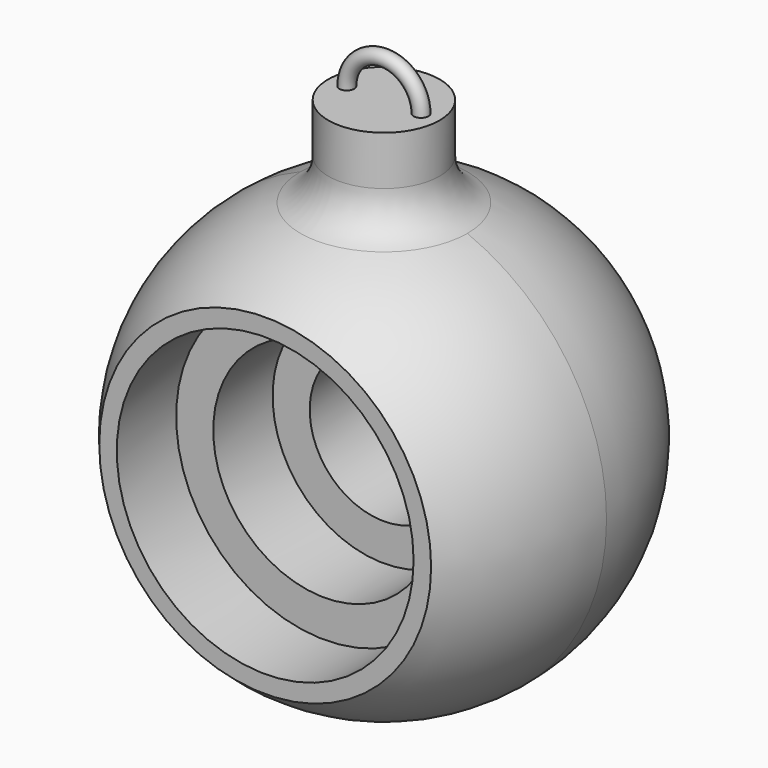
from build123d import *

# Parameters (mm, degrees)
F3_R      = 6.35
F4_DEPTH  = 63.5
F3_R_2    = 12.7
F5_DEPTH  = 50.8
F3_R_3    = 19.05
F6_DEPTH  = 38.1
F3_R_4    = 25.4
F7_DEPTH  = 25.4
F3_R_5    = 31.75
F8_DEPTH  = 12.7
F10_R     = 9.525
F11_DEPTH = 12.7
F14_R     = 1.27


# Not quite as in the source:
# - a fillet or chamfer that OpenCascade refuses, or shapes differently, is made with other operations: its cross-section is extruded or revolved along the edge and cut away or added


with BuildPart() as f1:
    # F0 (on Top) → F1 (revolve)
    with BuildSketch(Plane.XY):
        with BuildLine():
            ThreePointArc((0, -38.1), (26.9407683632, -26.9407683632), (38.1, 0))
            ThreePointArc((38.1, 0), (26.9407683632, 26.9407683632), (0, 38.1))
            Line((0, 38.1), (0, -38.1))
        make_face()
    revolve(axis=Axis((0, 0, 0), (0, 1, 0)))

    # F3 (on offset) → F4 (cut)
    with BuildSketch(Plane.XZ.offset(38.1)):
        Circle(F3_R)
    extrude(amount=-F4_DEPTH, mode=Mode.SUBTRACT)

    # F3 (on offset) → F5 (cut)
    with BuildSketch(Plane.XZ.offset(38.1)):
        Circle(F3_R_2)
        Circle(F3_R, mode=Mode.SUBTRACT)
    extrude(amount=-F5_DEPTH, mode=Mode.SUBTRACT)

    # F3 (on offset) → F6 (cut)
    with BuildSketch(Plane.XZ.offset(38.1)):
        Circle(F3_R_3)
        Circle(F3_R_2, mode=Mode.SUBTRACT)
    extrude(amount=-F6_DEPTH, mode=Mode.SUBTRACT)

    # F3 (on offset) → F7 (cut)
    with BuildSketch(Plane.XZ.offset(38.1)):
        Circle(F3_R_4)
        Circle(F3_R_3, mode=Mode.SUBTRACT)
    extrude(amount=-F7_DEPTH, mode=Mode.SUBTRACT)

    # F3 (on offset) → F8 (cut)
    with BuildSketch(Plane.XZ.offset(38.1)):
        Circle(F3_R_5)
        Circle(F3_R_4, mode=Mode.SUBTRACT)
    extrude(amount=-F8_DEPTH, mode=Mode.SUBTRACT)

    # F10 (on offset) → F11 (join, symmetric)
    with BuildSketch(Plane.XY.offset(38.1)):
        Circle(F10_R)
    extrude(amount=F11_DEPTH, both=True)

    # F12: fillet of radius 7.62 on 1 edges, made by hand

    # F12_s1 → F12_t2 (revolve)
    with BuildSketch(Plane.XZ):
        with BuildLine():
            ThreePointArc((14.2875000004, 35.3196452948), (10.8268297748, 38.1238648566), (9.5250000004, 42.3835743538))
            Line((9.5250000004, 42.3835743538), (9.525, 36.8901663726))
            ThreePointArc((9.525, 36.8901663726), (11.9321172967, 36.1833466781), (14.2875000004, 35.3196452948))
        make_face()
    revolve(axis=Axis((2e-10, 0, 36.8901663726), (0, 0, 1)))

    # F15: sweep along a path in F13
    with BuildLine(Plane.XZ) as f15_path:
        ThreePointArc((6.35, 50.8), (0, 57.15), (-6.35, 50.8))
    # F14 (on face) → F15 (sweep)
    with BuildSketch(Plane.XY.offset(50.8)):
        with Locations((-6.35, 0)):
            Circle(F14_R)
    sweep(path=f15_path.line)


solid = f1.part
